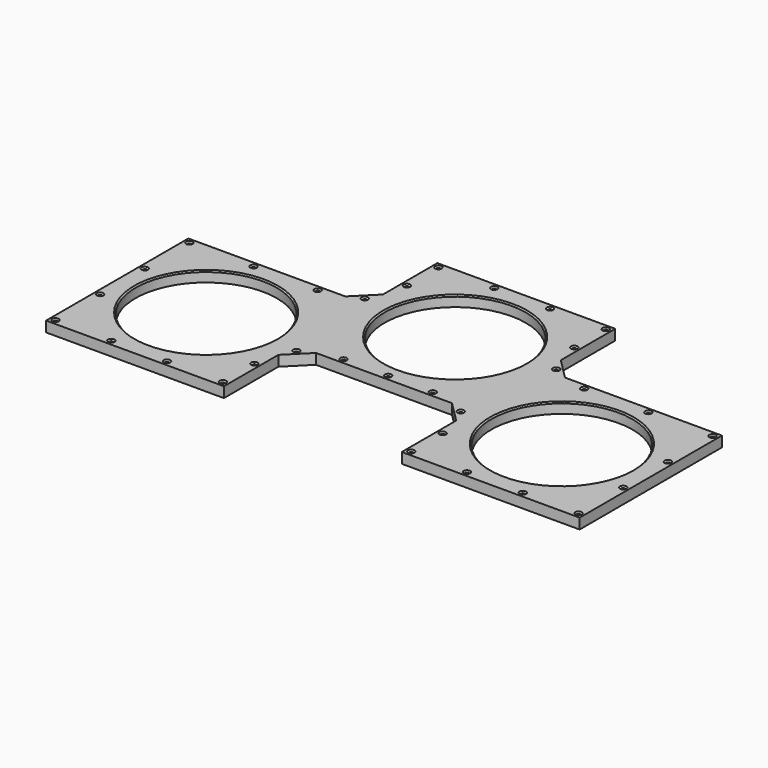
from build123d import *

# Parameters (mm, degrees)
F0_R           = 85.725
F1_DEPTH       = 12.7
F3_D           = 4.7625
F3_CSINK_D     = 7.9375
F3_CSINK_ANGLE = 85
F4_SIZE        = 1.5875


# Not quite as in the source:
# - a feature names something its author has since deleted; it is built from what else it names


with BuildPart() as f1:
    # F0 (on Top) → F1 (new body)
    with BuildSketch(Plane.XY):
        Polygon((-107.95, 133.35), (-133.35, 107.95), (-323.85, 107.95), (-323.85, -107.95), (-107.95, -107.95), (-107.95, -25.4), (-82.55, 0), (82.55, 0), (107.95, -25.4), (107.95, -107.95), (323.85, -107.95), (323.85, 107.95), (133.35, 107.95), (107.95, 133.35), (107.95, 215.9), (-107.95, 215.9), align=None)
        with Locations((-215.9, 0)):
            Circle(F0_R, mode=Mode.SUBTRACT)
        with Locations((215.9, 0)):
            Circle(F0_R, mode=Mode.SUBTRACT)
        with Locations((0, 107.95)):
            Circle(F0_R, mode=Mode.SUBTRACT)
    extrude(amount=F1_DEPTH)

    # F3 (through all)
    with Locations(Plane.XY.offset(12.7)):
        with Locations((-239.6099832965, 101.6), (-161.7199665929, 101.6), (-116.1598719395, 116.1598719395), (-101.6, 161.7199665929), (-101.6, 209.55), (-33.8666666667, 209.55), (33.8666666667, 209.55), (101.6, 209.55), (101.6, 161.7199665929), (116.1598719395, 116.1598719395), (161.7199665929, 101.6), (239.6099832965, 101.6), (317.5, 33.8666666667), (317.5, 101.6), (317.5, -33.8666666667), (317.5, -101.6), (249.7666666667, -101.6), (182.0333333333, -101.6), (114.3, -53.7699665929), (114.3, -101.6), (99.7401280605, -8.2098719395), (54.1800334071, 6.35), (0, 6.35), (-54.1800334071, 6.35), (-99.7401280605, -8.2098719395), (-114.3, -53.7699665929), (-114.3, -101.6), (-182.0333333333, -101.6), (-249.7666666667, -101.6), (-317.5, -101.6), (-317.5, -33.8666666667), (-317.5, 33.8666666667), (-317.5, 101.6)):
            CounterSinkHole(F3_D / 2, F3_CSINK_D / 2, counter_sink_angle=F3_CSINK_ANGLE)

    # F4
    f4_edges = [f1.edges().sort_by_distance(p)[0] for p in [
        (-85.725, 107.95, 12.7),
        (-301.625, 0, 12.7),
        (130.175, 0, 12.7),
    ]]
    chamfer(f4_edges, length=F4_SIZE)


solid = f1.part
